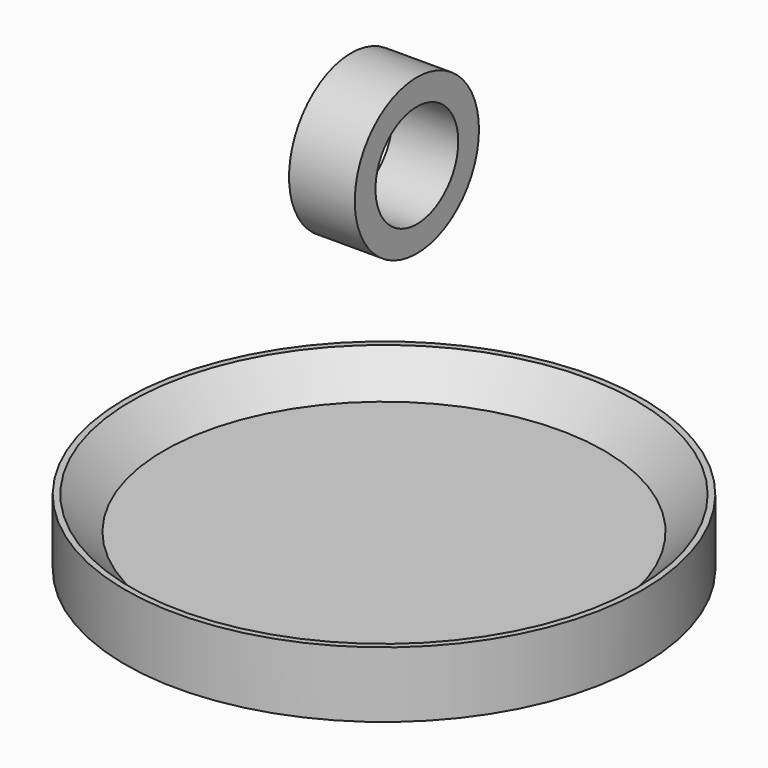
from build123d import *

# Parameters (mm, degrees)
F0_R     = 50
F1_DEPTH = 6.35
F2_R     = 50
F2_R_2   = 42.5
F3_DEPTH = 6.35
F4_SIZE  = 6.34999
F5_R     = 15
F5_R_2   = 10
F6_DEPTH = 6.35


# Not quite as in the source:
# - a fillet or chamfer is up to 0.001 mm smaller than in the source, because OpenCascade refuses the exact size


with BuildPart() as f1:
    # F0 (on Top) → F1 (new body)
    with BuildSketch(Plane.XY):
        Circle(F0_R)
    extrude(amount=F1_DEPTH)

    # F2 (on face) → F3 (join)
    with BuildSketch(Plane.XY.offset(6.35)):
        Circle(F2_R)
        Circle(F2_R_2, mode=Mode.SUBTRACT)
    extrude(amount=F3_DEPTH)

    # F4 (size 6.35 in the source; OpenCascade refuses exactly that, so slightly less here)
    f4_edges = [f1.edges().sort_by_distance(p)[0] for p in [
        (-42.5, 0, 12.7),
    ]]
    chamfer(f4_edges, length=F4_SIZE)


with BuildPart() as f6:
    # F5 (on Right) → F6 (new body, symmetric)
    with BuildSketch(Plane.YZ):
        with Locations((0, 70.7316364521)):
            Circle(F5_R)
        with Locations((0, 70.7316364521)):
            Circle(F5_R_2, mode=Mode.SUBTRACT)
    extrude(amount=F6_DEPTH, both=True)


solid = Compound([f1.part, f6.part])
